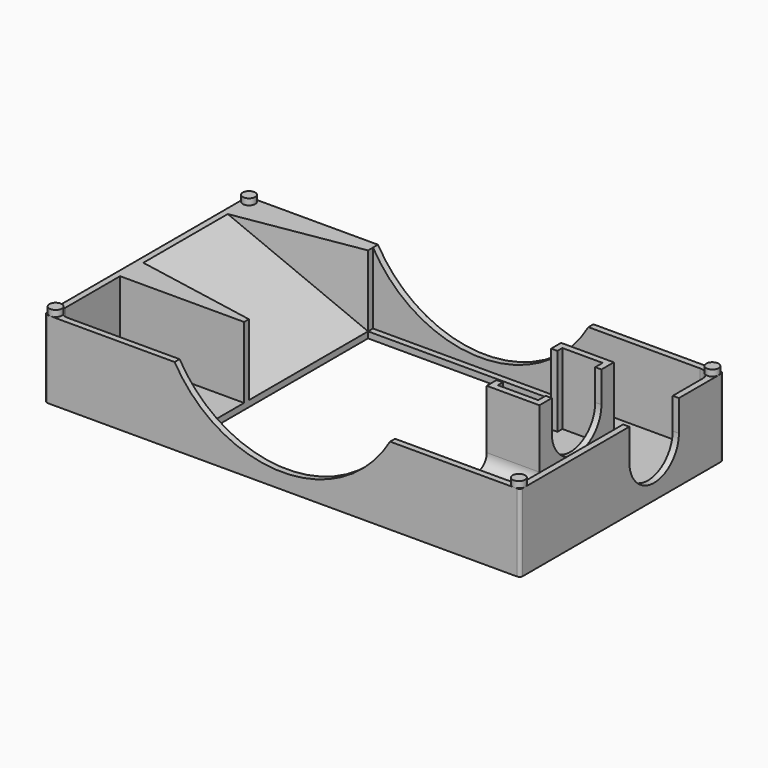
from build123d import *

# Parameters (mm, degrees)
F0_W         = 153.5
F0_H         = 82
F1_DEPTH     = 25
F2_W         = 149.5
F2_H         = 78
F3_DEPTH     = 23
F5_DEPTH     = 50
F6_W         = 40
F6_H         = 2
F7_DEPTH     = 23
F8_W         = 69.5
F8_H         = 74
F9_DEPTH     = 2.001
F12_DEPTH    = 25
F14_W        = 2
F14_H        = 26
F14_H_2      = 2
F15_DEPTH    = 23
F17_DEPTH    = 27.001
F19_DEPTH    = 82.001
F20_R        = 2
F21_DEPTH    = 2
F22_T1_DEPTH = 23
F22_T3_DEPTH = 17
F23_R        = 1


# Not quite as in the source:
# - a fillet or chamfer that OpenCascade refuses, or shapes differently, is made with other operations: its cross-section is extruded or revolved along the edge and cut away or added


with BuildPart() as f1:
    # F0 (on Top) → F1 (new body)
    with BuildSketch(Plane.XY):
        Rectangle(F0_W, F0_H)
    extrude(amount=F1_DEPTH)

    # F2 (on face) → F3 (cut)
    with BuildSketch(Plane.XY.offset(25)):
        Rectangle(F2_W, F2_H)
    extrude(amount=-F3_DEPTH, mode=Mode.SUBTRACT)

    # F4 (on face) → F5 (join)
    with BuildSketch(Plane.XZ.offset(-39)):
        Polygon((-34.75, 2), (-74.75, 25), (-74.75, 2), align=None)
    extrude(amount=F5_DEPTH)

    # F6 (on face) → F7 (join)
    with BuildSketch(Plane.XY.offset(2)):
        with Locations((-54.75, -12)):
            Rectangle(F6_W, F6_H)
    extrude(amount=F7_DEPTH)

    # F8 (on face) → F9 (cut, through all)
    with BuildSketch(Plane.XY.offset(2)):
        Rectangle(F8_W, F8_H)
    extrude(amount=-F9_DEPTH, mode=Mode.SUBTRACT)

    # F11 (on face) → F12 (join)
    with BuildSketch(Plane.XY.offset(25)):
        Polygon((-74.75, 39), (-74.75, 30.4142603609), (-34.75, 37), (-34.75, 39), align=None)
        Polygon((-74.75, -11), (-35.1230073053, -11), (-35.1229473745, -10.9961439342), (-74.75, -3.6334587345), align=None)
    extrude(amount=-F12_DEPTH)

    # F14 (on face) → F15 (join)
    with BuildSketch(Plane.XY.offset(2)):
        Polygon((36.75, 26), (49.75, 26), (51.75, 26), (51.75, 28), (34.75, 28), (34.75, 26), align=None)
        with Locations((50.75, 13)):
            Rectangle(F14_W, F14_H)
        Polygon((51.75, 0), (49.75, 0), (36.75, 0), (34.75, 0), (34.75, -2), (51.75, -2), align=None)
        with Locations((35.75, 25)):
            Rectangle(F14_W, F14_H_2)
        with Locations((35.75, 1)):
            Rectangle(F14_W, F14_H_2)
    extrude(amount=F15_DEPTH)

    # F16 (on face) → F17 (cut, through all)
    with BuildSketch(Plane(origin=(49.75, 0, 0), x_dir=(0, -1, 0), z_dir=(-1, 0, 0))):
        with BuildLine():
            Line((-3, 25), (-23, 25))
            Line((-23, 25), (-23, 15))
            ThreePointArc((-23, 15), (-13.0980438814, 4.9995097688), (-3, 14.8019609728))
            Line((-3, 14.8019609728), (-3, 25))
        make_face()
    extrude(amount=-F17_DEPTH, mode=Mode.SUBTRACT)

    # F18 (on face) → F19 (cut, through all)
    with BuildSketch(Plane.XZ.offset(41)):
        with BuildLine():
            Line((34.75, 25), (-34.75, 25))
            ThreePointArc((-34.75, 25), (0, 5), (34.75, 25))
        make_face()
    extrude(amount=-F19_DEPTH, mode=Mode.SUBTRACT)

    # F20 (on face) → F21 (join)
    with BuildSketch(Plane.XY.offset(25)):
        with Locations((-74.75, 39)):
            Circle(F20_R)
        with Locations((74.75, 39)):
            Circle(F20_R)
        with Locations((-74.75, -39)):
            Circle(F20_R)
        with Locations((74.75, -39)):
            Circle(F20_R)
    extrude(amount=F21_DEPTH)

    # F22: fillet of radius 4 on 5 edges, made by hand

    # F22_s2 → F22_t1 (join)
    with BuildSketch(Plane.XY.offset(2)):
        with BuildLine():
            ThreePointArc((-70.75, -39), (-73.5784271247, -37.8284271247), (-74.75, -35))
            Line((-74.75, -35), (-74.75, -39))
            Line((-74.75, -39), (-70.75, -39))
        make_face()
        with BuildLine():
            ThreePointArc((74.75, 35), (73.5784271247, 37.8284271247), (70.75, 39))
            Line((70.75, 39), (74.75, 39))
            Line((74.75, 39), (74.75, 35))
        make_face()
        with BuildLine():
            ThreePointArc((70.75, -39), (73.5784271247, -37.8284271247), (74.75, -35))
            Line((74.75, -35), (74.75, -39))
            Line((74.75, -39), (70.75, -39))
        make_face()
    extrude(amount=F22_T1_DEPTH)

    # F22_s4 → F22_t3 (join)
    with BuildSketch(Plane.YZ.offset(34.75)):
        with BuildLine():
            ThreePointArc((-6, 2), (-3.1715728753, 3.1715728753), (-2, 6))
            Line((-2, 6), (-2, 2))
            Line((-2, 2), (-6, 2))
        make_face()
        with BuildLine():
            ThreePointArc((32, 2), (29.1715728753, 3.1715728753), (28, 6))
            Line((28, 6), (28, 2))
            Line((28, 2), (32, 2))
        make_face()
    extrude(amount=F22_T3_DEPTH)

    # F23
    f23_edges = [f1.edges().sort_by_distance(p)[0] for p in [
        (76.75, -41, 12.5),
        (-76.75, -41, 12.5),
        (-76.75, 41, 12.5),
        (76.75, 41, 12.5),
    ]]
    fillet(f23_edges, radius=F23_R)


solid = f1.part
